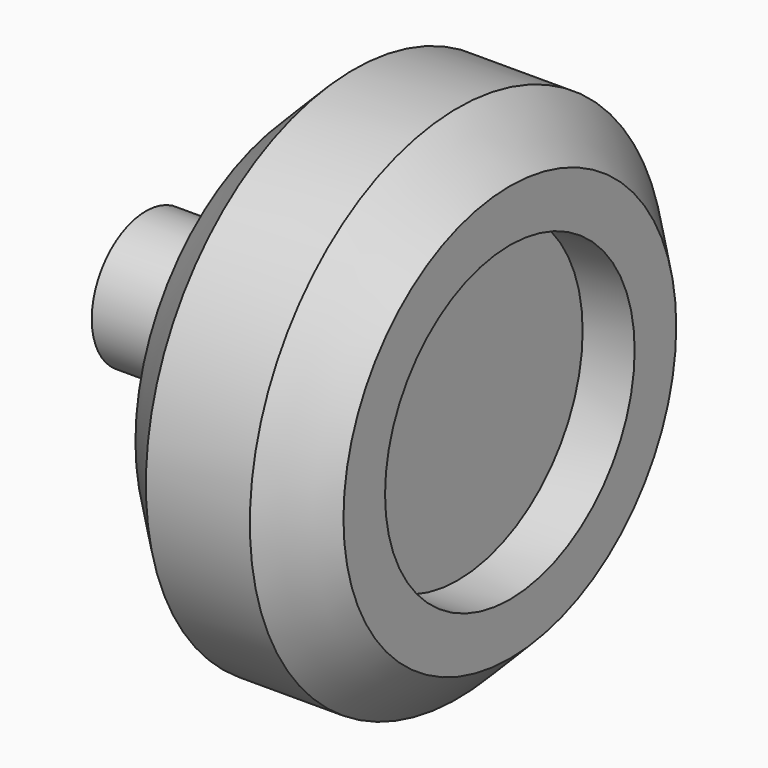
from build123d import *

# Parameters (mm, degrees)
F0_R     = 25
F1_DEPTH = 20
F2_SIZE  = 5
F3_SIZE  = 5
F4_R     = 15
F5_DEPTH = 5
F6_R     = 15
F7_DEPTH = 5
F8_R     = 6.5
F8_R_2   = 5
F9_DEPTH = 20
F10_T    = 2.5


# Not quite as in the source:
# - a shell that OpenCascade refuses in one call is made with other operations: the cavity is built on its own and cut out


with BuildPart() as f1:
    # F0 (on Right) → F1 (new body)
    with BuildSketch(Plane.YZ):
        Circle(F0_R)
    extrude(amount=F1_DEPTH)

    # F2
    f2_edges = [f1.edges().sort_by_distance(p)[0] for p in [
        (20, -25, 0),
    ]]
    chamfer(f2_edges, length=F2_SIZE)

    # F3
    f3_edges = [f1.edges().sort_by_distance(p)[0] for p in [
        (0, -25, 0),
    ]]
    chamfer(f3_edges, length=F3_SIZE)

    # F4 (on face) → F5 (cut)
    with BuildSketch(Plane(origin=(0, 0, 0), x_dir=(0, -1, 0), z_dir=(-1, 0, 0))):
        Circle(F4_R)
    extrude(amount=-F5_DEPTH, mode=Mode.SUBTRACT)

    # F6 (on face) → F7 (cut)
    with BuildSketch(Plane.YZ.offset(20)):
        Circle(F6_R)
    extrude(amount=-F7_DEPTH, mode=Mode.SUBTRACT)

    # F8 (on face) → F9 (join)
    with BuildSketch(Plane(origin=(5, 0, 0), x_dir=(0, -1, 0), z_dir=(-1, 0, 0))):
        Circle(F8_R)
        Circle(F8_R_2, mode=Mode.SUBTRACT)
    extrude(amount=F9_DEPTH)

    # F10: shell of thickness 2.5, made by hand


with BuildPart() as f10_core1:
    # F10_t2: copy of F1
    add(f1.part)

    # the walls: a layer under each face that stays
    f10_faces = [f10_core1.faces().sort_by_distance(p)[0] for p in [
        (10, -25, 0),
        (2.5, -22.5, 0),
        (17.5, -22.5, 0),
        (0, -13.3333333333, -13.3333333333),
        (20, -13.3333333333, -13.3333333333),
        (2.5, 15, 0),
        (17.5, -15, 0),
        (5, 10, -10),
        (15, 0, 0),
        (-5, 6.5, 0),
        (-5, 5, 0),
        (5, 0, 0),
    ]]
    thicken(f10_faces, amount=-F10_T, mode=Mode.SUBTRACT)

    # F10_s3 → F10_t4 (revolve, cut)
    with BuildSketch(Plane.XY):
        Polygon((4.975, -14.975), (5, -17.5), (7.5, -17.5), (7.5, -15), align=None)
    revolve(axis=Axis((5, 0, 0), (-1, 0, 0)), mode=Mode.SUBTRACT)

    # F10_s5 → F10_t6 (revolve, cut)
    with BuildSketch(Plane.XY):
        Polygon((15.025, 14.975), (15, 17.5), (12.5, 17.5), (12.5, 15), align=None)
    revolve(axis=Axis((15, 0, 0), (1, 0, 0)), mode=Mode.SUBTRACT)

    # F10_s7 → F10_t8 (revolve, cut)
    with BuildSketch(Plane.XY):
        Polygon((4.975, -6.525), (7.5, -6.5), (7.5, -4), (5, -4), align=None)
    revolve(axis=Axis((5, 0, 0), (-1, 0, 0)), mode=Mode.SUBTRACT)

    # F10_s9 → F10_t10 (revolve, cut)
    with BuildSketch(Plane.XY):
        Polygon((4.975, -4.975), (5, -7.5), (7.5, -7.5), (7.5, -5), align=None)
    revolve(axis=Axis((5, 0, 0), (-1, 0, 0)), mode=Mode.SUBTRACT)


with BuildPart() as f1_1:
    add(f1.part)

    # what is left inside the walls is the cavity
    f10_cavity = [f10_core1.part.solids().sort_by_distance(p)[0] for p in [
        (11.321489, -22.475, 0),
    ]]
    add(f10_cavity, mode=Mode.SUBTRACT)


solid = f1_1.part
